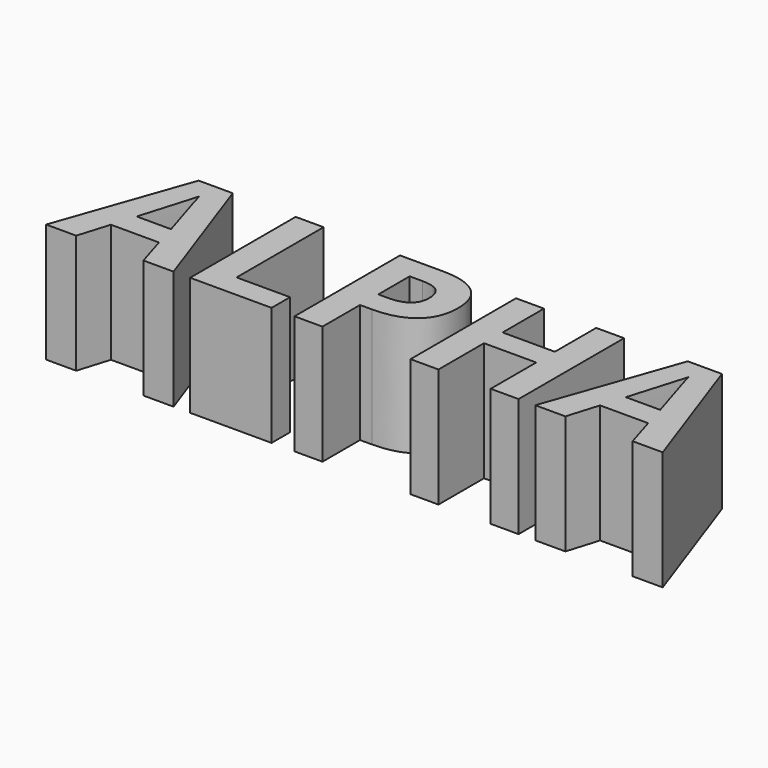
from build123d import *

# Parameters (mm, degrees)
F0_TEXT_SIZE = 39.453470769
F1_DEPTH     = 25.4
F2_W         = 4.9597955254
F2_H         = 12.7641654849
F3_DEPTH     = 10
F4_R         = 6


# Not quite as in the source:
# - Text() gives the source's letters only with a copy of the font that has no kerning and outlines rounded to 1/6400 em; it was checked with that copy


with BuildPart() as f1:
    # F0 (on Top) → F1 (new body)
    with BuildSketch(Plane.XY):
        with Locations((0, 0)):
            Text('ALPHA', F0_TEXT_SIZE, font='Open Sans', font_style=FontStyle.BOLD, text_align=(TextAlign.LEFT, TextAlign.BOTTOM))
    extrude(amount=F1_DEPTH)

    # F2 (on face) → F3 (join)
    with BuildSketch(Plane(origin=(0, 0, 0), x_dir=(-0.3316690168, -0.9433958147, 0), z_dir=(-0.9433958147, 0.3316690168, 0))):
        with Locations((-14.9901061757, 12.7)):
            Rectangle(F2_W, F2_H)
    extrude(amount=F3_DEPTH)

    # F4
    f4_edges = [f1.edges().sort_by_distance(p)[0] for p in [
        (-4.462204, 17.458294, 6.317917),
        (-4.462204, 17.458294, 19.082083),
    ]]
    fillet(f4_edges, radius=F4_R)


solid = f1.part
